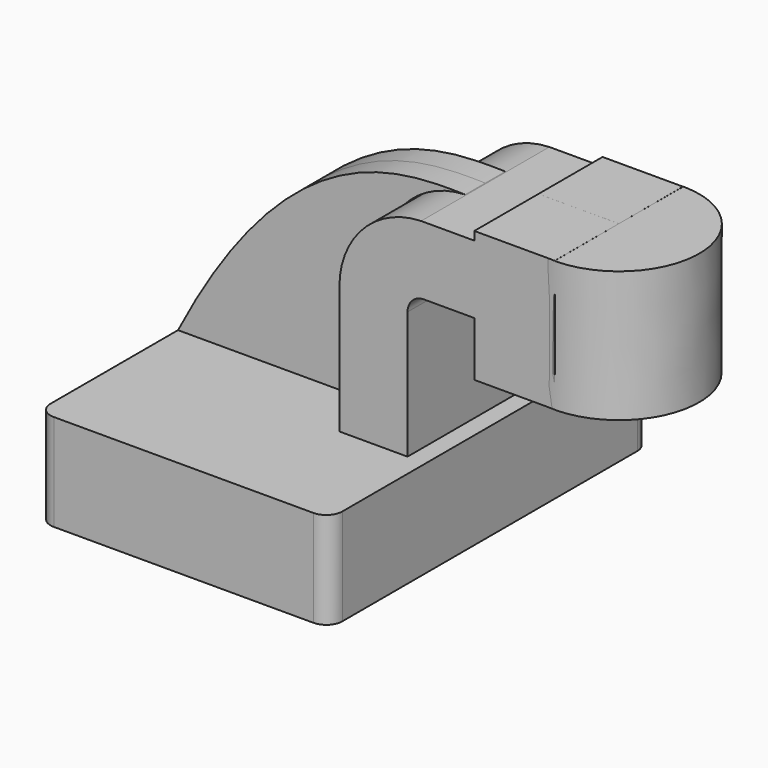
from build123d import *

# Parameters (mm, degrees)
F1_DEPTH = 63.5
F2_DEPTH = 25.4
F3_DEPTH = 7.9375
F5_R     = 5.08


# Not quite as in the source:
# - ends of sketch curves that miss each other by under 0.0002 mm in the source are joined


with BuildPart() as f1:
    # F0 (on Front) → F1 (new body, symmetric)
    with BuildSketch(Plane.XZ):
        Polygon((-42.4631357271, 15.3269270076), (-42.4631357271, -15.3269278245), (50.0009615827, -15.3269278245), (50.0009615827, 15.3269270076), (44.2532325515, 15.3269270076), (33.5852317512, 15.3269270076), (22.6632287853, 15.3269270076), (22.4044577503, 15.3269270076), align=None)
    extrude(amount=F1_DEPTH, both=True)

    # F0 (on Front) → F3 (join, symmetric)
    with BuildSketch(Plane.XZ):
        with BuildLine():
            add(Edge.make_bspline(
                [(-42.4631357271, 15.3269270076), (-7.3203722905, 83.1905780265), (26.4507513371, 83.1905752423), (48.56082653, 82.7370360494)],
                knots=[0, 0, 0, 0, 113.2673143763, 113.2673143763, 113.2673143763, 113.2673143763], degree=3))
            Line((-42.4631357271, 15.3269270076), (22.4044577503, 15.3269270076))
            Line((22.4044577503, 15.3269270076), (22.4044577503, 55.6962154806))
            ThreePointArc((22.4044577503, 55.6962154806), (30.0135223742, 74.5068614342), (48.56082653, 82.7370360494))
        make_face()
    extrude(amount=F3_DEPTH, both=True)

    # F5
    f5_edges = [f1.edges().sort_by_distance(p)[0] for p in [
        (-42.463136, -63.5, 0),
        (50.000962, -63.5, 0),
        (50.000962, 63.5, 0),
        (-42.463136, 63.5, 0),
    ]]
    fillet(f5_edges, radius=F5_R)


with BuildPart() as f2:
    # F0 (on Front) → F2 (new body, symmetric)
    with BuildSketch(Plane.XZ):
        with BuildLine():
            Line((33.5852317512, 15.3269270076), (44.2532325515, 15.3269270076))
            Line((44.2532325515, 15.3269270076), (44.2532325515, 55.6962154806))
            ThreePointArc((44.2532325515, 55.6962154806), (45.6414524036, 59.2359562846), (49.0658950772, 60.8882612482))
            Line((49.0658950772, 60.8882612482), (65.4116496444, 60.8882612482))
            Line((65.4116496444, 60.8882612482), (65.4116496444, 71.5562620485))
            Line((65.4116496444, 71.5562620485), (48.7713574063, 71.5562620485))
            ThreePointArc((48.7713574063, 71.5562620485), (37.9939440951, 66.6752806679), (33.5852317512, 55.6962154806))
            Line((33.5852317512, 55.6962154806), (33.5852317512, 15.3269270076))
        make_face()
        with BuildLine():
            Line((22.6632287853, 55.6962154806), (22.6632287853, 15.326927416))
            Line((22.6632287853, 15.326927416), (33.5852317512, 15.3269270076))
            Line((33.5852317512, 15.3269270076), (33.5852317512, 55.6962154806))
            ThreePointArc((33.5852317512, 55.6962154806), (37.9939440951, 66.6752806679), (48.7713574063, 71.5562620485))
            Line((48.7713574063, 71.5562620485), (65.4116496444, 71.5562620485))
            Line((65.4116496444, 71.5562620485), (65.4116496444, 82.4782650144))
            Line((65.4116496444, 82.4782650144), (48.565139174, 82.4782650144))
            ThreePointArc((48.565139174, 82.4782650144), (30.1980256678, 74.325407217), (22.6632287853, 55.6962154806))
        make_face()
        Polygon((65.4116496444, 85.1775221527), (65.4116496444, 82.7370360494), (65.4116496444, 82.4782650144), (65.4116496444, 71.5562620485), (65.4116496444, 60.8882612482), (65.4116496444, 43.6356849968), (90.872772038, 43.6356849968), (90.9117330309, 85.1775221527), align=None)
    extrude(amount=F2_DEPTH, both=True)


with BuildPart() as f4:
    # F0 (on Front) → F4 (revolve)
    with BuildSketch(Plane.XZ):
        Polygon((65.4116496444, 85.1775221527), (65.4116496444, 82.7370360494), (65.4116496444, 82.4782650144), (65.4116496444, 71.5562620485), (65.4116496444, 60.8882612482), (65.4116496444, 43.6356849968), (90.872772038, 43.6356849968), (90.9117330309, 85.1775221527), align=None)
    revolve(axis=Axis((90.8922525345, 0, 64.4066035748), (0.0009378732, 0, 0.9999995602)))


solid = Compound([f1.part, f2.part, f4.part])
